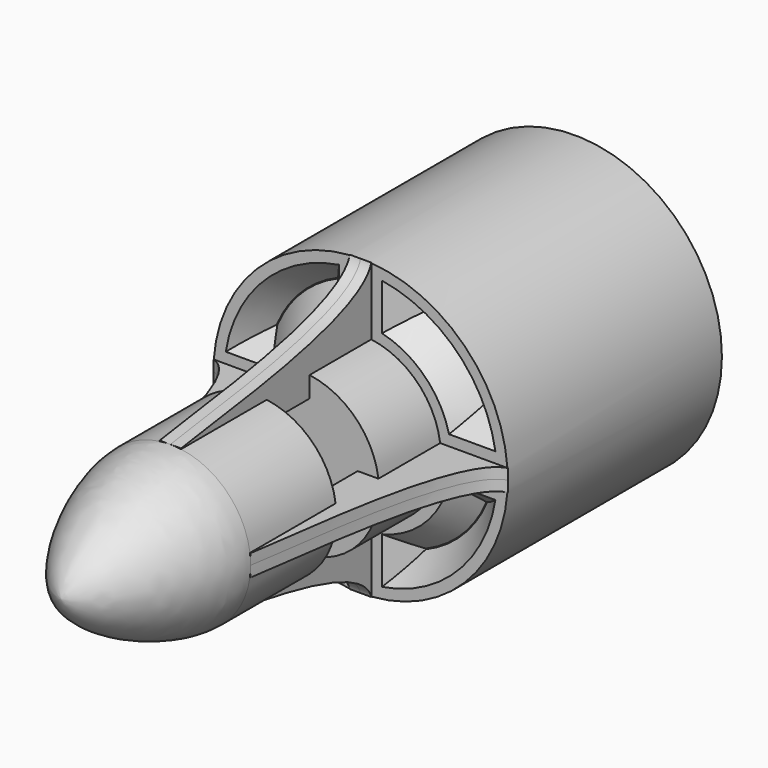
from build123d import *

# Parameters (mm, degrees)
F0_R                     = 27.5
F2_DEPTH                 = 50
F6_DEPTH                 = 2
F6_DEPTH_BACK            = 2
F7_COUNT                 = 4
F9_DEPTH                 = 5
DRAFT_F9_DRAFTED_ANGLE   = 40
DRAFT_F9_2_DRAFTED_ANGLE = 40
DRAFT_F9_3_DRAFTED_ANGLE = 40
DRAFT_F9_4_DRAFTED_ANGLE = 40


# Not quite as in the source:
# - an extrude with a draft is written as a straight extrude whose walls are then drafted


with BuildPart() as f2:
    # F0 (on Front) → F2 (new body)
    with BuildSketch(Plane.XZ):
        Circle(F0_R)
    extrude(amount=F2_DEPTH)

    # F3 (on Top) → F4 (revolve)
    with BuildSketch(Plane.XY):
        with BuildLine():
            Line((0, -120), (0, -50))
            Line((0, -50), (-15, -50))
            Line((-15, -50), (-15, -64.415422976))
            Line((-15, -64.415422976), (-3.9522200823, -64.415422976))
            Line((-3.9522200823, -64.415422976), (-3.9522200823, -74.415422976))
            Line((-3.9522200823, -74.415422976), (-15, -74.415422976))
            Line((-15, -74.415422976), (-15, -94.415422976))
            add(Edge.make_bspline(
                [(0, -120), (-6.8356664851, -118.8801941276), (-15, -103.0590899435), (-15, -94.415422976)],
                knots=[0, 0, 0, 0, 29.6575552178, 29.6575552178, 29.6575552178, 29.6575552178], degree=3))
        make_face()
    revolve(axis=Axis((0, -85, 0), (0, -1, 0)))

    # F5 (on Top) → F6 (join, two sides)
    with BuildSketch(Plane.XY) as f6_sk:
        with BuildLine():
            add(Edge.make_bspline(
                [(15, -94.415422976), (16.6003517807, -85.6350776553), (19.3110350519, -52.3280873895), (27.5, -50)],
                knots=[0, 0, 0, 0, 46.1408690657, 46.1408690657, 46.1408690657, 46.1408690657], degree=3))
            Line((27.5, -50), (11, -50))
            Line((11, -50), (11, -94.415422976))
            Line((11, -94.415422976), (15, -94.415422976))
        make_face()
    extrude(amount=F6_DEPTH)
    extrude(f6_sk.sketch, amount=-F6_DEPTH_BACK)

    # F7: F2 ×4 about axis
    f7_axis = Axis((0, 0, 0), (0, 1, 0))


with BuildPart() as f2_1:
    add(f2.part)
    for i in range(1, F7_COUNT):
        add(f2.part.rotate(f7_axis, i * 360 / F7_COUNT))


with BuildPart() as f9_drafted:
    # F8 (on face) → F9 (new body)
    with BuildSketch(Plane.XZ.offset(50)):
        with BuildLine():
            Line((25.1843205189, -4), (16.5227116419, -4))
            ThreePointArc((16.5227116419, -4), (12.0208152802, -12.0208152802), (4, -16.5227116419))
            Line((4, -16.5227116419), (4, -25.1843205189))
            ThreePointArc((4, -25.1843205189), (18.0312229203, -18.0312229203), (25.1843205189, -4))
        make_face()
    extrude(amount=-F9_DEPTH)

    # draft_F9_drafted
    draft_f9_drafted_walls = [f9_drafted.faces().sort_by_distance(p)[0] for p in [
        (4, -46.6666666667, -20.8535160804),
        (18.0312229203, -46.6666666667, -18.0312229203),
        (20.8535160804, -46.6666666667, -4),
        (12.0208152802, -46.6666666667, -12.0208152802),
    ]]
    draft(draft_f9_drafted_walls, neutral_plane=Plane(origin=(0, -50, 0), x_dir=(1, 0, 0), z_dir=(0, 1, 0)), angle=DRAFT_F9_DRAFTED_ANGLE)


with BuildPart() as f2_2:
    add(f2_1.part)

    # join_F9_drafted: cut F9_drafted
    add(f9_drafted.part, mode=Mode.SUBTRACT)


with BuildPart() as f9_2_drafted:
    # F8 (on face) → F9, piece 2 (new body)
    with BuildSketch(Plane.XZ.offset(50)):
        with BuildLine():
            Line((-4, -25.1843205189), (-4, -16.5227116419))
            ThreePointArc((-4, -16.5227116419), (-12.0208152802, -12.0208152802), (-16.5227116419, -4))
            Line((-16.5227116419, -4), (-25.1843205189, -4))
            ThreePointArc((-25.1843205189, -4), (-18.0312229203, -18.0312229203), (-4, -25.1843205189))
        make_face()
    extrude(amount=-F9_DEPTH)

    # draft_F9_2_drafted
    draft_f9_2_drafted_walls = [f9_2_drafted.faces().sort_by_distance(p)[0] for p in [
        (-20.8535160804, -46.6666666667, -4),
        (-18.0312229203, -46.6666666667, -18.0312229203),
        (-4, -46.6666666667, -20.8535160804),
        (-12.0208152802, -46.6666666667, -12.0208152802),
    ]]
    draft(draft_f9_2_drafted_walls, neutral_plane=Plane(origin=(0, -50, 0), x_dir=(1, 0, 0), z_dir=(0, 1, 0)), angle=DRAFT_F9_2_DRAFTED_ANGLE)


with BuildPart() as f2_3:
    add(f2_2.part)

    # join_F9_2_drafted: cut F9_2_drafted
    add(f9_2_drafted.part, mode=Mode.SUBTRACT)


with BuildPart() as f9_3_drafted:
    # F8 (on face) → F9, piece 3 (new body)
    with BuildSketch(Plane.XZ.offset(50)):
        with BuildLine():
            ThreePointArc((25.1843205189, 4), (18.0312229203, 18.0312229203), (4, 25.1843205189))
            Line((4, 25.1843205189), (4, 16.5227116419))
            ThreePointArc((4, 16.5227116419), (12.0208152802, 12.0208152802), (16.5227116419, 4))
            Line((16.5227116419, 4), (25.1843205189, 4))
        make_face()
    extrude(amount=-F9_DEPTH)

    # draft_F9_3_drafted
    draft_f9_3_drafted_walls = [f9_3_drafted.faces().sort_by_distance(p)[0] for p in [
        (20.8535160804, -46.6666666667, 4),
        (18.0312229203, -46.6666666667, 18.0312229203),
        (4, -46.6666666667, 20.8535160804),
        (12.0208152802, -46.6666666667, 12.0208152802),
    ]]
    draft(draft_f9_3_drafted_walls, neutral_plane=Plane(origin=(0, -50, 0), x_dir=(1, 0, 0), z_dir=(0, 1, 0)), angle=DRAFT_F9_3_DRAFTED_ANGLE)


with BuildPart() as f2_4:
    add(f2_3.part)

    # join_F9_3_drafted: cut F9_3_drafted
    add(f9_3_drafted.part, mode=Mode.SUBTRACT)


with BuildPart() as f9_4_drafted:
    # F8 (on face) → F9, piece 4 (new body)
    with BuildSketch(Plane.XZ.offset(50)):
        with BuildLine():
            Line((-25.1843205189, 4), (-16.5227116419, 4))
            ThreePointArc((-16.5227116419, 4), (-12.0208152802, 12.0208152802), (-4, 16.5227116419))
            Line((-4, 16.5227116419), (-4, 25.1843205189))
            ThreePointArc((-4, 25.1843205189), (-18.0312229203, 18.0312229203), (-25.1843205189, 4))
        make_face()
    extrude(amount=-F9_DEPTH)

    # draft_F9_4_drafted
    draft_f9_4_drafted_walls = [f9_4_drafted.faces().sort_by_distance(p)[0] for p in [
        (-4, -46.6666666667, 20.8535160804),
        (-18.0312229203, -46.6666666667, 18.0312229203),
        (-20.8535160804, -46.6666666667, 4),
        (-12.0208152802, -46.6666666667, 12.0208152802),
    ]]
    draft(draft_f9_4_drafted_walls, neutral_plane=Plane(origin=(0, -50, 0), x_dir=(1, 0, 0), z_dir=(0, 1, 0)), angle=DRAFT_F9_4_DRAFTED_ANGLE)


with BuildPart() as f2_5:
    add(f2_4.part)

    # join_F9_4_drafted: cut F9_4_drafted
    add(f9_4_drafted.part, mode=Mode.SUBTRACT)


solid = f2_5.part
